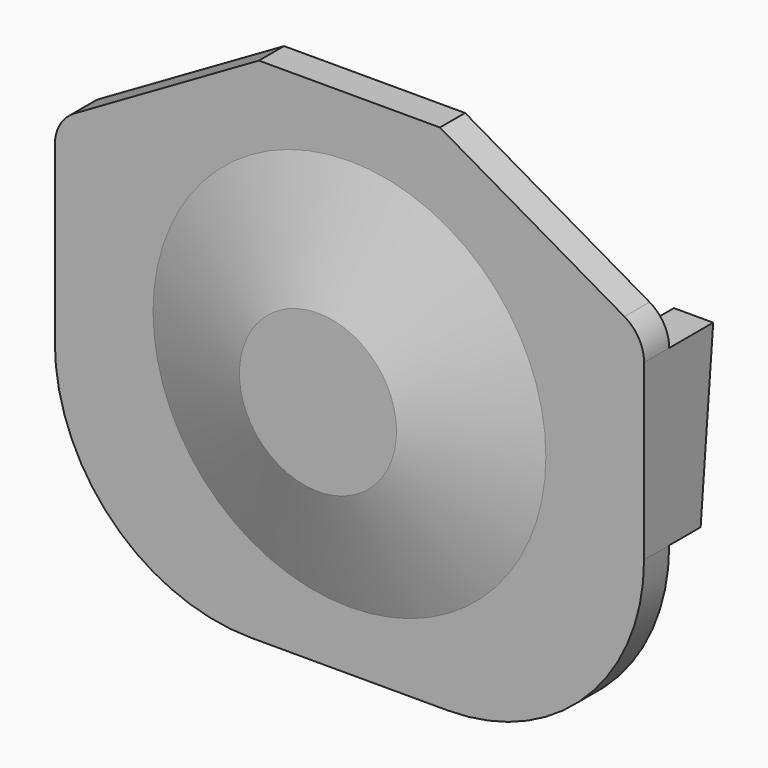
from build123d import *

# Parameters (mm, degrees)
F1_DEPTH = 0.8
F2_R     = 5
F3_R     = 1
F4_R     = 5
F5_DEPTH = 1
F6_SIZE2 = 2.99999
F6_SIZE  = 0.99999
F8_DEPTH = 1


# Not quite as in the source:
# - a fillet or chamfer is up to 0.001 mm smaller than in the source, because OpenCascade refuses the exact size


with BuildPart() as f1:
    # F0 (on Front) → F1 (new body)
    with BuildSketch(Plane.XZ):
        Polygon((7.5, 3.5), (2.3038475773, 6.5), (-2.3038475773, 6.5), (-7.5, 3.5), (-7.5, -6.5), (7.5, -6.5), align=None)
    extrude(amount=F1_DEPTH)

    # F2
    f2_edges = [f1.edges().sort_by_distance(p)[0] for p in [
        (7.5, -0.4, -6.5),
        (-7.5, -0.4, -6.5),
    ]]
    fillet(f2_edges, radius=F2_R)

    # F3
    f3_edges = [f1.edges().sort_by_distance(p)[0] for p in [
        (7.5, -0.4, 3.5),
        (-7.5, -0.4, 3.5),
    ]]
    fillet(f3_edges, radius=F3_R)

    # F4 (on face) → F5 (join)
    with BuildSketch(Plane.XZ.offset(0.8)):
        Circle(F4_R)
    extrude(amount=F5_DEPTH)

    # F6 (size 1 and 3 in the source; OpenCascade refuses exactly that, so slightly less here)
    f6_edges = [f1.edges().sort_by_distance(p)[0] for p in [
        (-5, -1.8, 0),
    ]]
    f6_side = f1.faces().sort_by_distance((-5, -1.3, 0))[0]
    chamfer(f6_edges, length=F6_SIZE, length2=F6_SIZE2, reference=f6_side)

    # F7 (on face) → F8 (join)
    with BuildSketch(Plane.YZ.offset(7.5)):
        Polygon((1.4, 2.9226497308), (0, 2.9226497308), (0, -1.5), (1, -1.5), align=None)
    extrude(amount=-F8_DEPTH)

    # F9: F1 across plane


with BuildPart() as f1_1:
    add(f1.part)
    add(f1.part.mirror(Plane.YZ))


solid = f1_1.part
